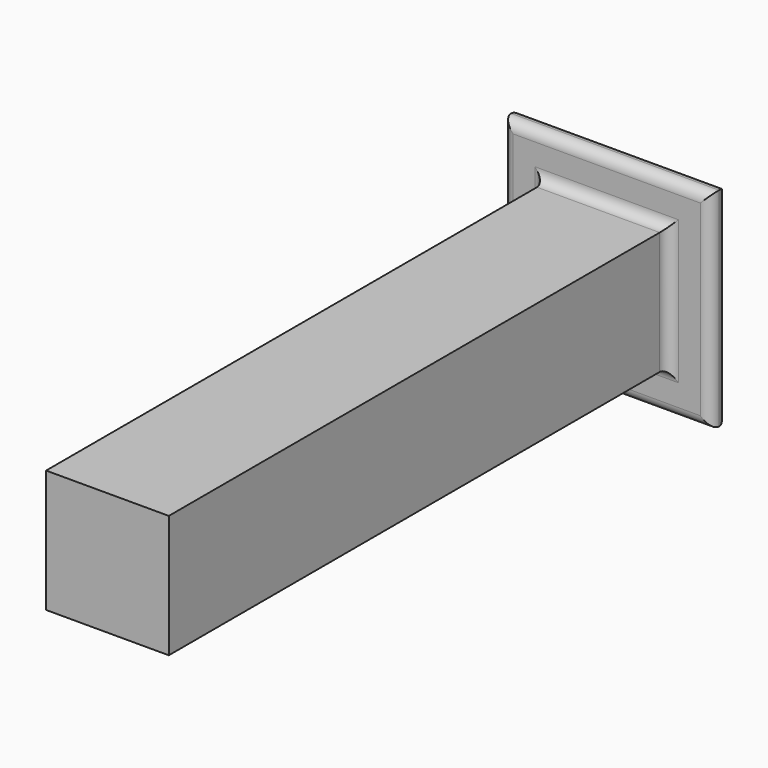
from build123d import *

# Parameters (mm, degrees)
F0_W     = 25.4
F0_H     = 25.4
F1_DEPTH = 2.54
F2_W     = 14.986
F2_H     = 14.986
F3_DEPTH = 76.2
F4_R     = 1.26999


# Not quite as in the source:
# - a fillet or chamfer is up to 0.001 mm smaller than in the source, because OpenCascade refuses the exact size


with BuildPart() as f1:
    # F0 (on Front) → F1 (new body)
    with BuildSketch(Plane.XZ):
        Rectangle(F0_W, F0_H)
    extrude(amount=F1_DEPTH)

    # F2 (on face) → F3 (join)
    with BuildSketch(Plane.XZ.offset(2.54)):
        Rectangle(F2_W, F2_H)
    extrude(amount=F3_DEPTH)

    # F4 (radius 1.27 in the source; OpenCascade refuses exactly that, so slightly less here)
    f4_edges = [f1.edges().sort_by_distance(p)[0] for p in [
        (0, 0, 12.7),
        (-12.7, 0, 0),
        (0, 0, -12.7),
        (12.7, 0, 0),
        (0, -2.54, 12.7),
        (12.7, -2.54, 0),
        (-12.7, -2.54, 0),
        (0, -2.54, -12.7),
        (0, -2.54, 7.493),
        (-7.493, -2.54, 0),
        (0, -2.54, -7.493),
        (7.493, -2.54, 0),
    ]]
    fillet(f4_edges, radius=F4_R)


solid = f1.part
